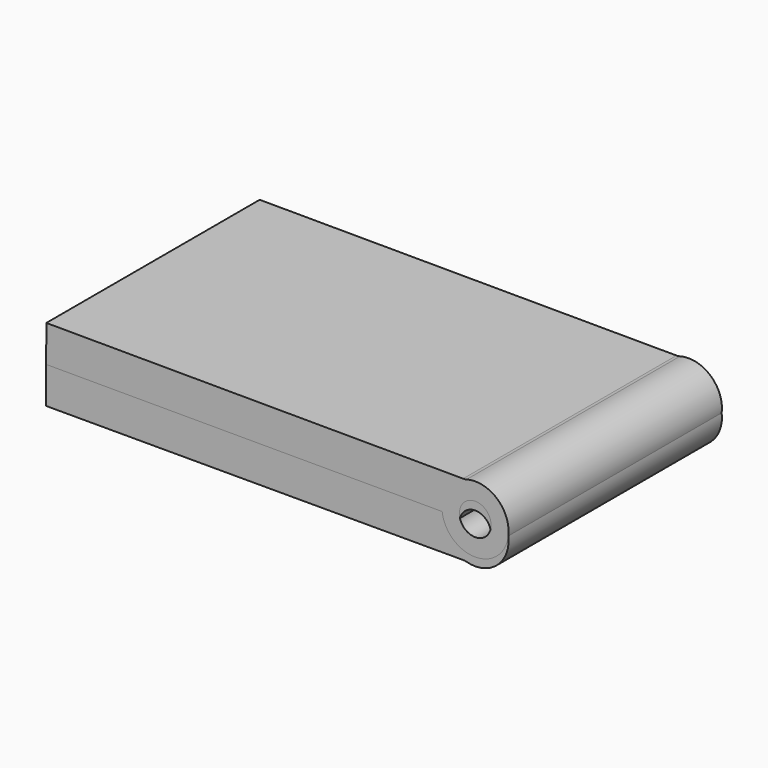
from build123d import *

# Parameters (mm, degrees)
F1_DEPTH    = 100
F2_T1_DEPTH = 100
F3_R        = 5.9375424291
F4_DEPTH    = 167.9


# Not quite as in the source:
# - a fillet or chamfer that OpenCascade refuses, or shapes differently, is made with other operations: its cross-section is extruded or revolved along the edge and cut away or added


with BuildPart() as f1:
    # F0 (on Front) → F1 (new body)
    with BuildSketch(Plane.XZ):
        with BuildLine():
            Line((-114.1351125863, -6.7254188471), (36.1845269799, -6.7254188471))
            Line((36.1845269799, -6.7254188471), (42.8799907786, -6.7254188471))
            ThreePointArc((42.8799907786, -6.7254188471), (57.28511127, 11.8717971065), (34.3334955709, 6.7155121653))
            Line((34.3334955709, 6.7155121653), (-114.1748427859, 6.9940946996))
            Line((-114.1748427859, 6.9940946996), (-114.1351125863, 0.2745811529))
            Line((-114.1351125863, 0.2745811529), (-114.1351125863, -6.7254188471))
        make_face()
    extrude(amount=F1_DEPTH)

    # F2: fillet of radius 5 on 1 edges, made by hand

    # F2_s2 → F2_t1 (join)
    with BuildSketch(Plane.XZ):
        with BuildLine():
            add(Edge.make_bspline(
                [(43.4655953072, -6.8996803378), (42.8229343795, -6.7254188471), (42.1570664233, -6.7254188471)],
                knots=[0, 0, 0, 1, 1, 1], degree=2, weights=[1, 1, 1]))
            Line((42.1570664233, -6.7254188471), (42.8799907786, -6.7254188471))
            ThreePointArc((42.8799907786, -6.7254188471), (43.1717281765, -6.8161280686), (43.4655953072, -6.8996803378))
        make_face()
    extrude(amount=F2_T1_DEPTH)

    # F3 (on face) → F4 (cut)
    with BuildSketch(Plane.XZ.offset(100)):
        with Locations((46.7369175169, 5.1646659355)):
            Circle(F3_R)
    extrude(amount=-F4_DEPTH, mode=Mode.SUBTRACT)


with BuildPart() as f5_1:
    # F5: instance of F1
    add(f1.part.mirror(Plane(origin=(-39.9206736075, -50, 6.8548034325), x_dir=(1, 0, 0), z_dir=(0.001875868, 0, 0.9999982406))))


solid = Compound([f1.part, f5_1.part])
